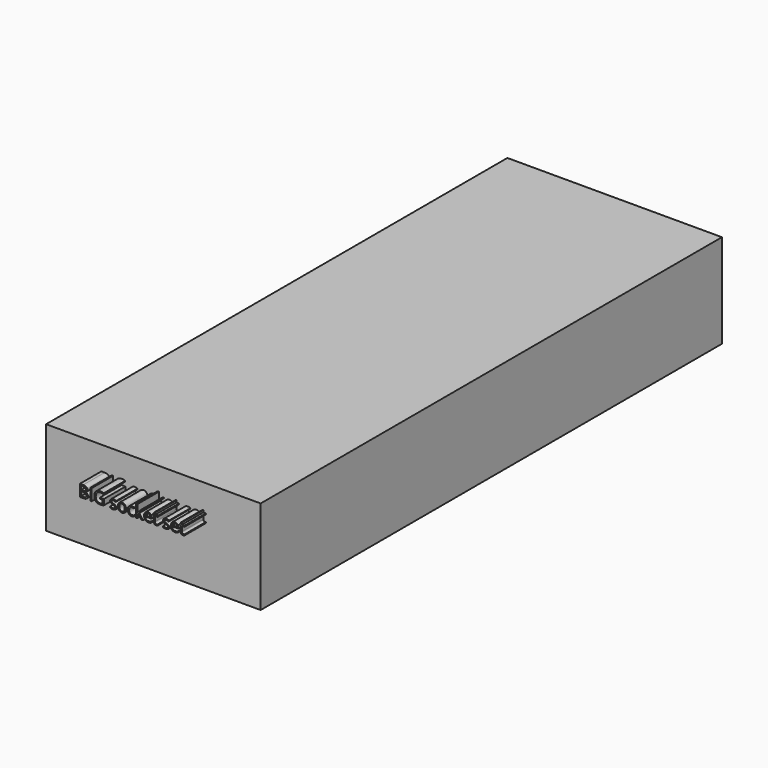
from build123d import *

# Parameters (mm, degrees)
F0_W         = 203.2
F0_H         = 88.9
F1_DEPTH     = 546.1
F2_TEXT_SIZE = 15.3811945594
F3_DEPTH     = 25.4


# Not quite as in the source:
# - Text() gives the source's letters only with a copy of the font that has no kerning and outlines rounded to 1/6400 em; it was checked with that copy


with BuildPart() as f1:
    # F0 (on Front) → F1 (new body)
    with BuildSketch(Plane.XZ):
        Rectangle(F0_W, F0_H)
    extrude(amount=F1_DEPTH)

    # F2 (on face) → F3 (join)
    with BuildSketch(Plane.XZ.offset(546.1)):
        with Locations((-50.8, 11.1351250473)):
            Text('BIG socket set', F2_TEXT_SIZE, font='Open Sans', text_align=(TextAlign.LEFT, TextAlign.BOTTOM))
    extrude(amount=F3_DEPTH)


solid = f1.part
